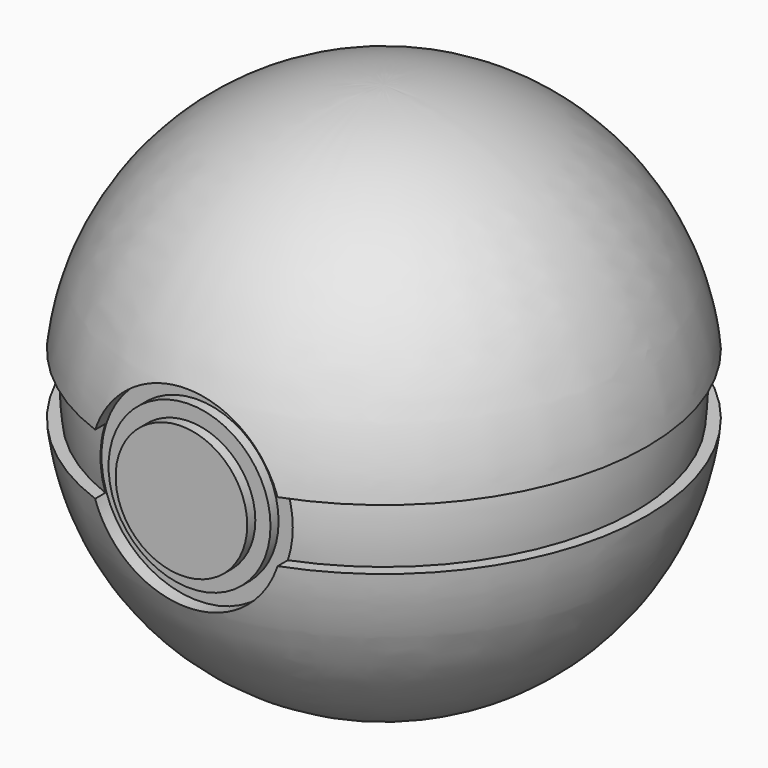
from build123d import *

# Parameters (mm, degrees)
F5_R      = 9.5
F6_DEPTH  = 20
F7_R      = 8
F8_DEPTH  = 1
F9_R      = 6.5
F10_DEPTH = 2


# Not quite as in the source:
# - ends of sketch curves that miss each other by under 0.0002 mm in the source are joined
# - a pattern or mirror of a feature is missing from the dataset's text; its kind, count and spacing are read off the source's solid


with BuildPart() as f1:
    # F0 (on Front) → F1 (revolve)
    with BuildSketch(Plane.XZ):
        with BuildLine():
            Line((0, 25), (0, -24.9999989992))
            ThreePointArc((0, -24.9999989992), (25.0000020016, 0), (0, 25))
        make_face()
    revolve(axis=Axis((0, 0, 5.004e-07), (0, 0, 1)))

    # F2 (on Front) → F3 (revolve)
    with BuildSketch(Plane.XZ):
        with BuildLine():
            Line((0, -3), (0, -26))
            ThreePointArc((0, -26), (17.4005104893, -19.4744901184), (26, -3))
            Line((26, -3), (0, -3))
        make_face()
    f3 = revolve(axis=Axis((0, 0, -14.5), (0, 0, 1)))

    # F3_copies: F3 across plane
    add(f3.mirror(Plane(origin=(0, 0, 3.2e-05), x_dir=(0, 1, -1e-05), z_dir=(-9e-06, 1e-05, 1))))

    # F5 (on offset) → F6 (cut)
    with BuildSketch(Plane.XZ.offset(23)):
        Circle(F5_R)
    extrude(amount=F6_DEPTH, mode=Mode.SUBTRACT)

    # F7 (on offset) → F8 (join)
    with BuildSketch(Plane.XZ.offset(23)):
        Circle(F7_R)
    extrude(amount=F8_DEPTH)

    # F9 (on offset) → F10 (join)
    with BuildSketch(Plane.XZ.offset(23)):
        Circle(F9_R)
    extrude(amount=F10_DEPTH)


solid = f1.part
